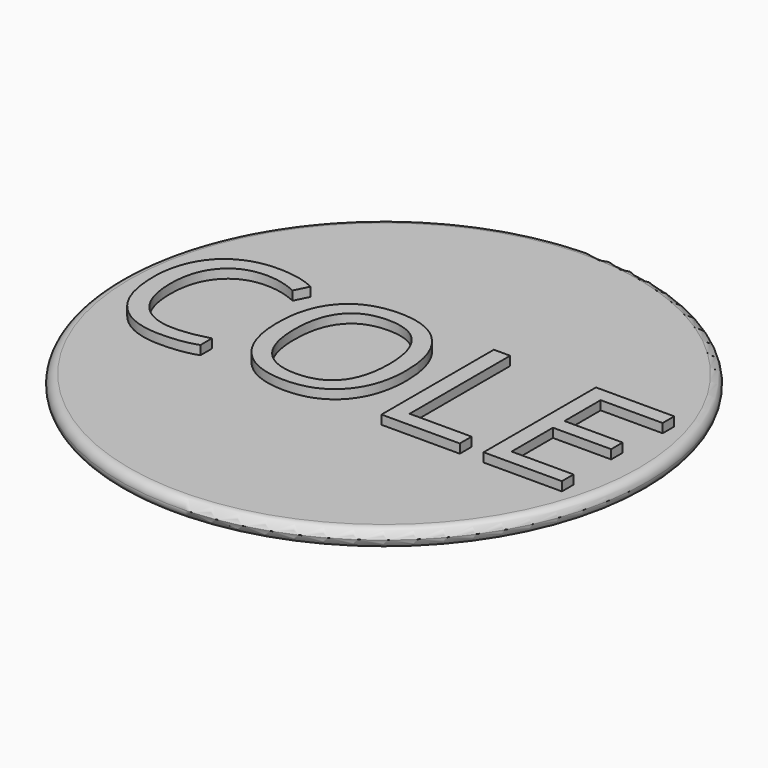
from build123d import *

# Parameters (mm, degrees)
F0_R         = 74.2564604032
F1_DEPTH     = 5.08
F2_R         = 2.54
F3_R         = 2.53999
F4_TEXT_SIZE = 55.3409171168
F5_DEPTH     = 2.54


# Not quite as in the source:
# - a fillet or chamfer is up to 0.001 mm smaller than in the source, because OpenCascade refuses the exact size
# - Text() gives the source's letters only with a copy of the font that has no kerning and outlines rounded to 1/6400 em; it was checked with that copy


with BuildPart() as f1:
    # F0 (on Top) → F1 (new body)
    with BuildSketch(Plane.XY):
        Circle(F0_R)
    extrude(amount=F1_DEPTH)

    # F2
    f2_edges = [f1.edges().sort_by_distance(p)[0] for p in [
        (-74.25646, 0, 5.08),
    ]]
    fillet(f2_edges, radius=F2_R)

    # F3 (radius 2.54 in the source; OpenCascade refuses exactly that, so slightly less here)
    f3_edges = [f1.edges().sort_by_distance(p)[0] for p in [
        (74.25646, 0, 1.27),
        (-74.25646, 0, 2.54),
        (-74.25646, 0, 0),
    ]]
    fillet(f3_edges, radius=F3_R)

    # F4 (on face) → F5 (join)
    with BuildSketch(Plane.XY.offset(5.08)):
        with Locations((-68.7164357992, -19.3198143218)):
            Text('COLE', F4_TEXT_SIZE, font='Open Sans', text_align=(TextAlign.LEFT, TextAlign.BOTTOM))
    extrude(amount=F5_DEPTH)


solid = f1.part
